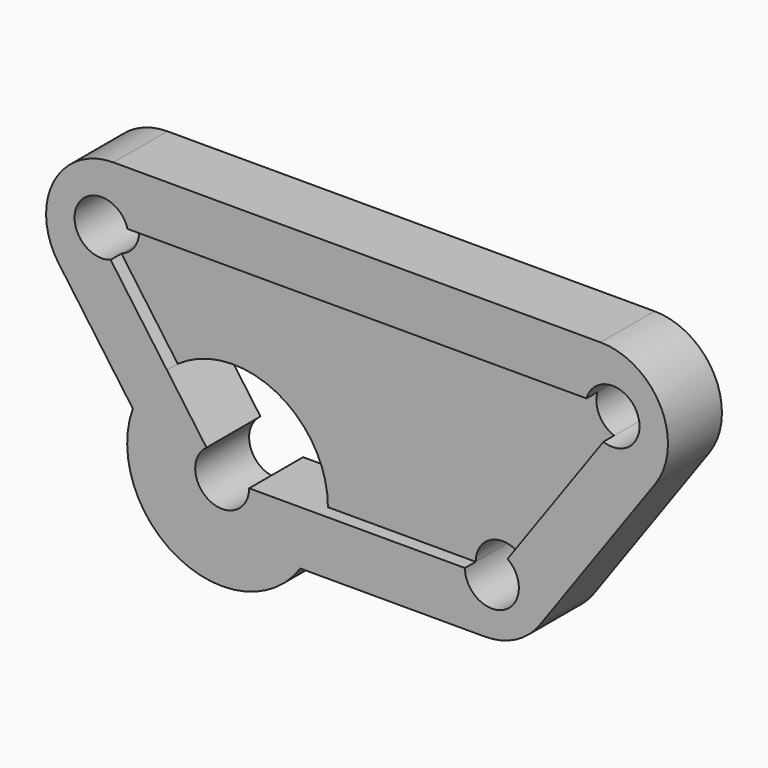
from build123d import *

# Parameters (mm, degrees)
F1_DEPTH = 15.875
F2_DEPTH = 9.525


with BuildPart() as f1:
    # F0 (on Front) → F1 (new body, symmetric)
    with BuildSketch(Plane.XZ):
        with BuildLine():
            ThreePointArc((174.448603, 46.228389), (169.051038, 35.837795), (157.44633, 34.279311))
            Line((157.44633, 34.279311), (112.323365, -28.892839))
            ThreePointArc((112.323365, -28.892839), (116.234069, -33.415968), (117.64164, -39.227254))
            ThreePointArc((117.64164, -39.227254), (104.94164, -51.927254), (92.24164, -39.227254))
            Line((92.24164, -39.227254), (22.665694, -39.227254))
            ThreePointArc((22.665694, -39.227254), (20.641741, -52.529225), (14.753065, -64.627254))
            Line((14.753065, -64.627254), (101.673817, -64.627254))
            ThreePointArc((101.673817, -64.627254), (116.202032, -61.108327), (127.509854, -51.331567))
            Line((127.509854, -51.331567), (181.938426, 24.868433))
            ThreePointArc((181.938426, 24.868433), (184.333461, 57.850961), (156.102388, 75.072746))
            Line((156.102388, 75.072746), (-73.219107, 75.072746))
            ThreePointArc((-73.219107, 75.072746), (-101.45018, 57.850961), (-99.055145, 24.868433))
            Line((-99.055145, 24.868433), (-64.123396, -24.036016))
            ThreePointArc((-64.123396, -24.036016), (-57.701548, -12.212367), (-48.053688, -2.833794))
            Line((-48.053688, -2.833794), (-74.563049, 34.279311))
            ThreePointArc((-74.563049, 34.279311), (-90.157751, 52.039675), (-66.641313, 49.672746))
            Line((-66.641313, 49.672746), (149.524593, 49.672746))
            ThreePointArc((149.524593, 49.672746), (163.487148, 58.808828), (174.448603, 46.228389))
        make_face()
        with BuildLine():
            ThreePointArc((14.753065, -64.627254), (20.641741, -52.529225), (22.665694, -39.227254))
            Line((22.665694, -39.227254), (-9.35836, -39.227254))
            ThreePointArc((-9.35836, -39.227254), (-27.869646, -50.519683), (-29.440085, -28.892839))
            Line((-29.440085, -28.892839), (-48.053688, -2.833794))
            ThreePointArc((-48.053688, -2.833794), (-57.701548, -12.212367), (-64.123396, -24.036016))
            Line((-64.123396, -24.036016), (-44.626574, -51.331567))
            ThreePointArc((-44.626574, -51.331567), (-33.318751, -61.108327), (-18.790536, -64.627254))
            Line((-18.790536, -64.627254), (14.753065, -64.627254))
        make_face()
        with BuildLine():
            ThreePointArc((-64.123396, -24.036016), (-42.523263, -78.994436), (14.753065, -64.627254))
            Line((14.753065, -64.627254), (-18.790536, -64.627254))
            ThreePointArc((-18.790536, -64.627254), (-33.318751, -61.108327), (-44.626574, -51.331567))
            Line((-44.626574, -51.331567), (-64.123396, -24.036016))
        make_face()
    extrude(amount=F1_DEPTH, both=True)

    # F0 (on Front) → F2 (join, symmetric)
    with BuildSketch(Plane.XZ):
        with BuildLine():
            Line((112.323365, -28.892839), (157.44633, 34.279311))
            ThreePointArc((157.44633, 34.279311), (150.456174, 40.417103), (149.524593, 49.672746))
            Line((149.524593, 49.672746), (-66.641313, 49.672746))
            ThreePointArc((-66.641313, 49.672746), (-66.284882, 47.966934), (-66.165322, 46.228389))
            ThreePointArc((-66.165322, 46.228389), (-68.474729, 38.925953), (-74.563049, 34.279311))
            Line((-74.563049, 34.279311), (-48.053688, -2.833794))
            ThreePointArc((-48.053688, -2.833794), (-1.593456, 0.539928), (22.665694, -39.227254))
            Line((22.665694, -39.227254), (92.24164, -39.227254))
            ThreePointArc((92.24164, -39.227254), (99.130354, -27.934825), (112.323365, -28.892839))
        make_face()
    extrude(amount=F2_DEPTH, both=True)


solid = f1.part
